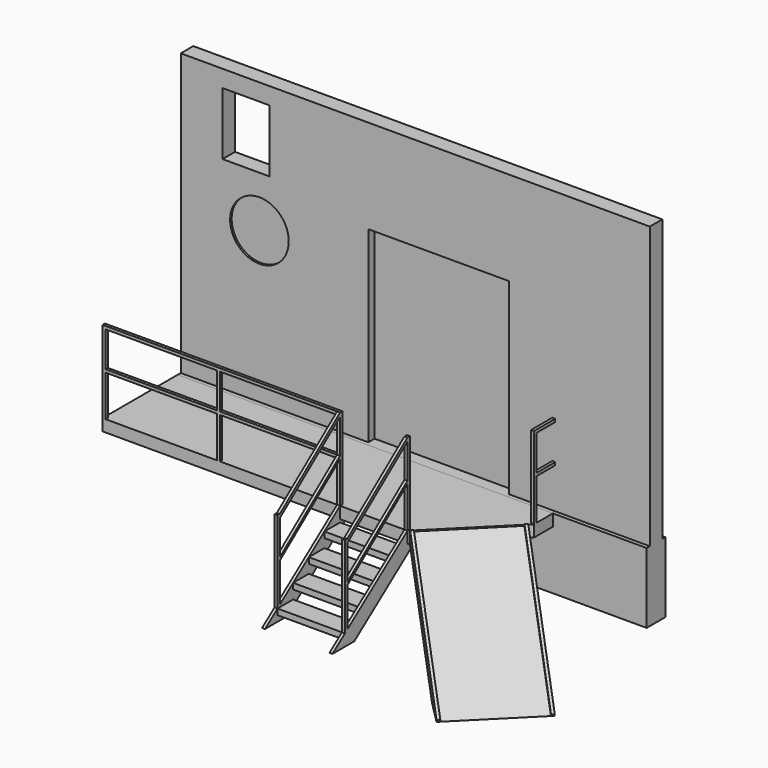
from build123d import *

# Parameters (mm, degrees)
F0_W      = 6096
F0_H      = 304.8
F1_DEPTH  = 914.4
F2_W      = 6096
F2_H      = 3657.6
F3_DEPTH  = 101.6
F5_W      = 1219.2
F5_H      = 152.4
F6_DEPTH  = 4876.8
F7_W      = 1828.8
F7_H      = 2438.4
F8_DEPTH  = 101.6
F9_SIZE   = 914.4
F12_W     = 254
F12_H     = 76.2
F13_DEPTH = 38.1
F14_DEPTH = 914.4
F15_W     = 254
F15_H     = 76.2
F16_DEPTH = 38.1
F17_W     = 38.1
F17_H     = 38.1
F18_DEPTH = 1066.8
F19_W     = 38.1
F19_H     = 38.1
F20_DEPTH = 3048
F21_W     = 38.1
F21_H     = 38.1
F22_DEPTH = 304.8
F23_W     = 38.1
F23_H     = 38.1
F24_DEPTH = 1066.8
F26_DEPTH = 38.1
F28_DEPTH = 38.1
F32_DEPTH = 38.1
F34_DEPTH = 25.4
F35_DEPTH = 1168.4
F37_DEPTH = 38.1
F38_R     = 381
F39_DEPTH = 25.4
F40_W     = 609.6
F40_H     = 812.8
F41_DEPTH = 254.001


with BuildPart() as f1:
    # F0 (on Top) → F1 (new body)
    with BuildSketch(Plane.XY):
        Rectangle(F0_W, F0_H)
    extrude(amount=F1_DEPTH)

    # F2 (on Front) → F3 (join, symmetric)
    with BuildSketch(Plane.XZ):
        with Locations((0, 2743.2)):
            Rectangle(F2_W, F2_H)
    extrude(amount=F3_DEPTH, both=True)

    # F7 (on face) → F8 (cut)
    with BuildSketch(Plane.XZ.offset(101.6)):
        with Locations((304.8, 2133.6)):
            Rectangle(F7_W, F7_H)
    extrude(amount=-F8_DEPTH, mode=Mode.SUBTRACT)

    # F38 (on face) → F39 (cut)
    with BuildSketch(Plane.XZ.offset(101.6)):
        with Locations((-2025.563955307, 2876.3597011566)):
            Circle(F38_R)
    extrude(amount=-F39_DEPTH, mode=Mode.SUBTRACT)

    # F40 (on face) → F41 (cut, through all)
    with BuildSketch(Plane.XZ.offset(101.6)):
        with Locations((-2200.0251152039, 3944.7877754211)):
            Rectangle(F40_W, F40_H)
    extrude(amount=-F41_DEPTH, mode=Mode.SUBTRACT)


with BuildPart() as f6:
    # F5 (on offset) → F6 (new body)
    with BuildSketch(Plane.YZ.offset(1828.8)):
        with Locations((-762, 838.2)):
            Rectangle(F5_W, F5_H)
    extrude(amount=-F6_DEPTH)

    # F9
    f9_edges = [f6.edges().sort_by_distance(p)[0] for p in [
        (1828.8, -1371.6, 838.2),
    ]]
    chamfer(f9_edges, length=F9_SIZE)

    # F12 (on plane+point) → F13 (join)
    with BuildSketch(Plane.YZ.offset(914.4)):
        Polygon((-2235.2, 0), (-2133.6, 76.2), (-2387.6, 76.2), (-2387.6, 152.4), (-2590.8, 0), align=None)
        with Locations((-2260.6, 114.3)):
            Rectangle(F12_W, F12_H)
        Polygon((-2133.6, 76.2), (-1879.6, 266.7), (-2133.6, 266.7), (-2133.6, 342.9), (-2387.6, 152.4), (-2133.6, 152.4), align=None)
        with Locations((-2006.6, 304.8)):
            Rectangle(F12_W, F12_H)
        Polygon((-1879.6, 266.7), (-1625.6, 457.2), (-1879.6, 457.2), (-1879.6, 533.4), (-2133.6, 342.9), (-1879.6, 342.9), align=None)
        with Locations((-1752.6, 495.3)):
            Rectangle(F12_W, F12_H)
        Polygon((-1625.6, 457.2), (-1371.6, 647.7), (-1625.6, 647.7), (-1625.6, 723.9), (-1879.6, 533.4), (-1625.6, 533.4), align=None)
        with Locations((-1498.6, 685.8)):
            Rectangle(F12_W, F12_H)
        Polygon((-1371.6, 647.7), (-1219.2, 762), (-1371.6, 762), (-1371.6, 914.4), (-1625.6, 723.9), (-1371.6, 723.9), align=None)
    extrude(amount=-F13_DEPTH)

    # F12 (on plane+point) → F14 (join)
    with BuildSketch(Plane.YZ.offset(914.4)):
        with Locations((-2260.6, 114.3)):
            Rectangle(F12_W, F12_H)
        with Locations((-2006.6, 304.8)):
            Rectangle(F12_W, F12_H)
        with Locations((-1752.6, 495.3)):
            Rectangle(F12_W, F12_H)
        with Locations((-1498.6, 685.8)):
            Rectangle(F12_W, F12_H)
    extrude(amount=-F14_DEPTH)

    # F15 (on face) → F16 (join)
    with BuildSketch(Plane(origin=(0, 0, 0), x_dir=(0, -1, 0), z_dir=(-1, 0, 0))):
        Polygon((1371.6, 914.4), (1371.6, 762), (1219.2, 762), (1371.6, 647.7), (1371.6, 723.9), (1625.6, 723.9), align=None)
        with Locations((1498.6, 685.8)):
            Rectangle(F15_W, F15_H)
        Polygon((2590.8, 0), (1625.6, 723.9), (1625.6, 647.7), (1371.6, 647.7), (2235.2, 0), align=None)
    extrude(amount=-F16_DEPTH)

    # F17 (on face) → F18 (join)
    with BuildSketch(Plane.XY.offset(914.4)):
        with Locations((-3028.95, -1352.55)):
            Rectangle(F17_W, F17_H)
        with Locations((-1543.05, -1352.55)):
            Rectangle(F17_W, F17_H)
        with Locations((19.05, -1352.55)):
            Rectangle(F17_W, F17_H)
        with Locations((895.35, -1352.55)):
            Rectangle(F17_W, F17_H)
        with Locations((1809.75, -438.15)):
            Rectangle(F17_W, F17_H)
    extrude(amount=F18_DEPTH)

    # F19 (on face) → F20 (join, through all)
    with BuildSketch(Plane(origin=(0, 0, 0), x_dir=(0, -1, 0), z_dir=(-1, 0, 0))):
        with Locations((1352.55, 1962.15)):
            Rectangle(F19_W, F19_H)
        with Locations((1352.55, 1466.85)):
            Rectangle(F19_W, F19_H)
    extrude(amount=F20_DEPTH)

    # F21 (on face) → F22 (join)
    with BuildSketch(Plane(origin=(0, -419.1, 0), x_dir=(-1, 0, 0), z_dir=(0, 1, 0))):
        with Locations((-1809.75, 1962.15)):
            Rectangle(F21_W, F21_H)
        with Locations((-1809.75, 1466.85)):
            Rectangle(F21_W, F21_H)
    extrude(amount=F22_DEPTH)

    # F23 (on face) → F24 (join)
    with BuildSketch(Plane.XY.offset(152.4)):
        with Locations((19.05, -2368.55)):
            Rectangle(F23_W, F23_H)
        with Locations((895.35, -2368.55)):
            Rectangle(F23_W, F23_H)
    extrude(amount=F24_DEPTH)

    # F25 (on face) → F26 (join)
    with BuildSketch(Plane(origin=(0, 0, 0), x_dir=(0, -1, 0), z_dir=(-1, 0, 0))):
        Polygon((2349.5, 1219.2), (1371.6, 1981.2), (1371.6, 1932.8988007302), (2349.5, 1170.8988007302), align=None)
        Polygon((2349.5, 723.9), (1371.6, 1485.9), (1371.6, 1447.8), (2349.5, 685.8), align=None)
    extrude(amount=-F26_DEPTH)

    # F27 (on face) → F28 (join)
    with BuildSketch(Plane.YZ.offset(914.4)):
        Polygon((-1371.6, 1981.2), (-2349.5, 1219.2), (-2349.5, 1170.8988007302), (-1371.6, 1932.8988007302), align=None)
        Polygon((-1371.6, 1485.9), (-2349.5, 723.9), (-2349.5, 685.8), (-1371.6, 1447.8), align=None)
    extrude(amount=-F28_DEPTH)


with BuildPart() as f32:
    # F31 (on face) → F32 (new body)
    with BuildSketch(Plane(origin=(640.8987193947, 640.8987193947, 0), x_dir=(-0.7071067812, 0.7071067812, 0), z_dir=(0.7071067812, 0.7071067812, 0))):
        Polygon((-1641.8461017924, 762), (-1641.8461017924, 914.4), (-4080.2461017924, 0), (-3673.8461017924, 0), align=None)
    extrude(amount=-F32_DEPTH)

    # F34 (add): a face of the model
    f34_faces = [f32.faces().sort_by_distance(p)[0] for p in [
        (2650.4934350778, -1395.6367646517, 457.2),
    ]]
    extrude(f34_faces, amount=F34_DEPTH)

    # F33 (on face) → F35 (join)
    with BuildSketch(Plane(origin=(613.9579510314, 613.9579510314, 0), x_dir=(0.7071067812, -0.7071067812, 0), z_dir=(-0.7071067812, -0.7071067812, 0))):
        Polygon((1641.8461017924, 914.4), (1641.8461017924, 873.7091821629), (3971.7372542269, 0), (4080.2461017924, 0), align=None)
    extrude(amount=F35_DEPTH)

    # F36 (on face) → F37 (join)
    with BuildSketch(Plane(origin=(-212.2256121069, -212.2256121069, 0), x_dir=(0.7071067812, -0.7071067812, 0), z_dir=(-0.7071067812, -0.7071067812, 0))):
        Polygon((3673.8461017924, 0), (3971.7372542269, 0), (1641.8461017924, 873.7091821629), (1641.8461017924, 762), align=None)
        Polygon((3971.7372542269, 0), (4080.2461017924, 0), (1641.8461017924, 914.4), (1641.8461017924, 873.7091821629), align=None)
        Polygon((4080.2461017924, 0), (4089.1646372088, 23.7827611103), (1650.7646372088, 938.1827611103), (1641.8461017924, 914.4), align=None)
    extrude(amount=-F37_DEPTH)


solid = Compound([f1.part, f6.part, f32.part])
